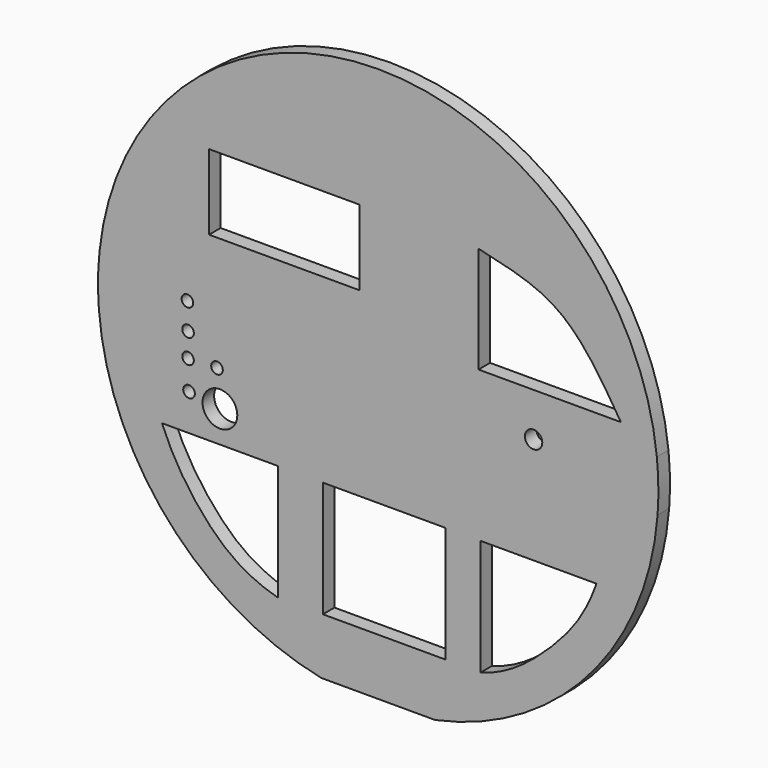
from build123d import *

# Parameters (mm, degrees)
F0_R     = 6
F0_R_2   = 2
F0_W     = 42.228937149
F0_H     = 40
F0_R_3   = 3
F0_W_2   = 52
F0_H_2   = 26
F1_DEPTH = 5


# Not quite as in the source:
# - the program builds the solid bodies; features that only make, move or delete a surface that nothing else refers to are left out


with BuildPart() as f1:
    # F0 (on Front) → F1 (new body)
    with BuildSketch(Plane.XZ):
        with BuildLine():
            Line((114.488999566, 5.1368772984), (153.7277594005, 5.1368772984))
            ThreePointArc((153.7277594005, 5.1368772984), (206.6891166454, 35.9273670532), (230.521004176, 92.3631780006))
            Line((230.521004176, 92.3631780006), (37.6957547904, 92.3631780006))
            ThreePointArc((37.6957547904, 92.3631780006), (61.527642321, 35.9273670532), (114.488999566, 5.1368772984))
        make_face()
        with BuildLine():
            add(Edge.make_bspline(
                [(59.4798011976, 64.6672644662), (63.1085559726, 55.6081011891), (73.7513924788, 39.0135130084), (88.0385711789, 27.8172641993), (99.4798011976, 24.6672644662)],
                knots=[0, 0, 0, 0, 0.4955592973, 1, 1, 1, 1], degree=3))
            Line((59.4798011976, 64.6672644662), (99.4798011976, 64.6672644662))
            Line((99.4798011976, 64.6672644662), (99.4798011976, 24.6672644662))
        make_face(mode=Mode.SUBTRACT)
        with Locations((79.4798011976, 75.4959482996)):
            Circle(F0_R, mode=Mode.SUBTRACT)
        with Locations((68.8243359327, 77.2860795259)):
            Circle(F0_R_2, mode=Mode.SUBTRACT)
        with Locations((68.4796720743, 87.2811824083)):
            Circle(F0_R_2, mode=Mode.SUBTRACT)
        with Locations((78.4747824073, 87.6258462667)):
            Circle(F0_R_2, mode=Mode.SUBTRACT)
        with Locations((136.1386179924, 44.6672644662)):
            Rectangle(F0_W, F0_H, mode=Mode.SUBTRACT)
        with BuildLine():
            Line((169.434517622, 64.6672644662), (209.434517622, 64.6672644662))
            add(Edge.make_bspline(
                [(169.434517622, 24.6672644662), (179.2577588513, 27.1916796699), (196.3345264834, 41.3050241265), (205.696706141, 54.1838165912), (209.434517622, 64.6672644662)],
                knots=[0, 0, 0, 0, 0.5114020852, 1, 1, 1, 1], degree=3))
            Line((169.434517622, 24.6672644662), (169.434517622, 64.6672644662))
        make_face(mode=Mode.SUBTRACT)
        with BuildLine():
            Line((37.6957547904, 92.3631780006), (230.521004176, 92.3631780006))
            ThreePointArc((230.521004176, 92.3631780006), (230.8000531475, 101.1758471342), (230.2752492915, 109.9773007924))
            Line((230.2752492915, 109.9773007924), (37.941509675, 109.9773007924))
            ThreePointArc((37.941509675, 109.9773007924), (37.4167058189, 101.1758471342), (37.6957547904, 92.3631780006))
        make_face()
        with Locations((68.4796720743, 95.552995801)):
            Circle(F0_R_2, mode=Mode.SUBTRACT)
        with Locations((68.259306113, 104.66844666)):
            Circle(F0_R_2, mode=Mode.SUBTRACT)
        with Locations((187.7316534519, 101.4121994376)):
            Circle(F0_R_3, mode=Mode.SUBTRACT)
        with BuildLine():
            Line((37.941509675, 109.9773007924), (230.2752492915, 109.9773007924))
            ThreePointArc((230.2752492915, 109.9773007924), (134.1083794832, 196.5278747198), (37.941509675, 109.9773007924))
        make_face()
        with Locations((101.7344622612, 140.218708396)):
            Rectangle(F0_W_2, F0_H_2, mode=Mode.SUBTRACT)
        with BuildLine():
            Line((168.7307208776, 116.4853125811), (168.7307208776, 153.218708396))
            add(Edge.make_bspline(
                [(168.7307208776, 153.218708396), (178.5376432275, 150.9342291161), (199.0201954085, 146.7686018938), (211.3988850452, 126.7827873103), (217.8624719381, 116.4853125811)],
                knots=[0, 0, 0, 0, 0.4802466092, 1, 1, 1, 1], degree=3))
            Line((217.8624719381, 116.4853125811), (168.7307208776, 116.4853125811))
        make_face(mode=Mode.SUBTRACT)
    extrude(amount=-F1_DEPTH)


solid = f1.part
